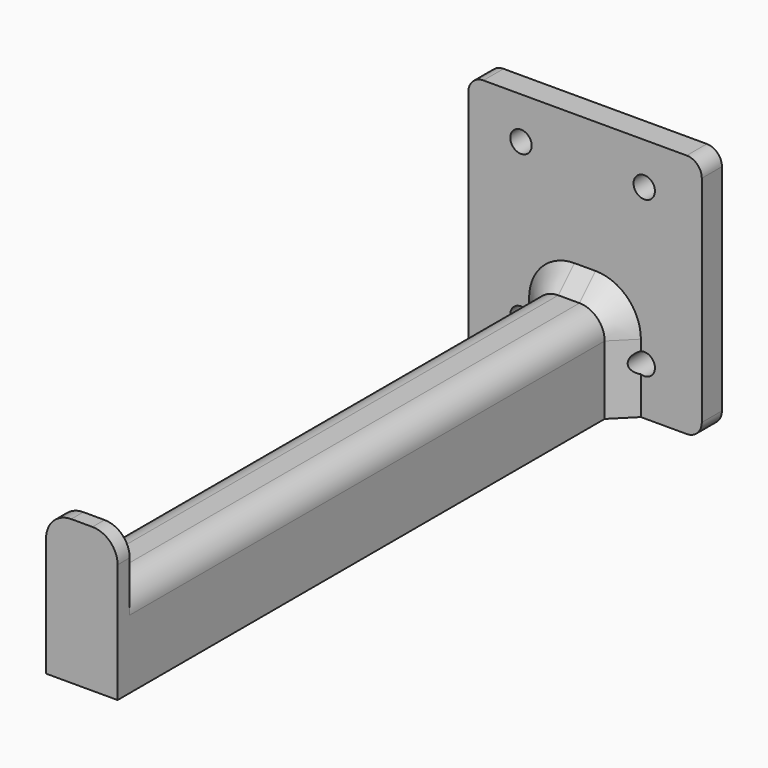
from build123d import *

# Parameters (mm, degrees)
F0_R         = 2.1251138046
F1_DEPTH     = 5
F0_W         = 14.2144468555
F0_H         = 18.6405025888
F2_DEPTH     = 130
F3_W         = 14.2144468555
F3_H         = 3
F4_DEPTH     = 10.03026
F5_R         = 5
F6_R         = 3
F7_T1_DEPTH  = 4.2144468555
F7_T6_DEPTH  = 13.6405025888
F7_S7_R      = 2.1251138046
F7_T8_DEPTH  = 9
F7_T10_ANGLE = 90
F7_T12_ANGLE = 90
F7_T16_DEPTH = 13.6405025888
F7_S17_R     = 2.1251138046
F7_T18_DEPTH = 9


# Not quite as in the source:
# - a fillet or chamfer that OpenCascade refuses, or shapes differently, is made with other operations: its cross-section is extruded or revolved along the edge and cut away or added


with BuildPart() as f1:
    # F0 (on Front) → F1 (new body)
    with BuildSketch(Plane.XZ):
        Polygon((16.5932904929, 31.273946166), (-29.8148933798, 31.273946166), (-29.8148933798, -17.4539741129), (-13.7278847396, -17.4539741129), (-13.7278847396, 1.186528476), (0.4865621158, 1.186528476), (0.4865621158, -17.4539741129), (16.5932904929, -17.4539741129), align=None)
        with Locations((-19.3455703557, -7.9430211366)):
            Circle(F0_R, mode=Mode.SUBTRACT)
        with Locations((5.1544296443, -7.9430211366)):
            Circle(F0_R, mode=Mode.SUBTRACT)
        with Locations((-19.3455703557, 22.9763388634)):
            Circle(F0_R, mode=Mode.SUBTRACT)
        with Locations((5.1544296443, 22.9763388634)):
            Circle(F0_R, mode=Mode.SUBTRACT)
    extrude(amount=F1_DEPTH)

    # F0 (on Front) → F2 (join)
    with BuildSketch(Plane.XZ):
        with Locations((-6.6206613119, -8.1337228185)):
            Rectangle(F0_W, F0_H)
    extrude(amount=F2_DEPTH)

    # F3 (on face) → F4 (join)
    with BuildSketch(Plane.XY.offset(1.186528476)):
        with Locations((-6.6206613119, -128.5)):
            Rectangle(F3_W, F3_H)
    extrude(amount=F4_DEPTH)

    # F5
    f5_edges = [f1.edges().sort_by_distance(p)[0] for p in [
        (0.486562, -66, 1.186528),
        (-13.727885, -66, 1.186528),
        (-13.727885, -128.5, 11.216788),
        (0.486562, -128.5, 11.216788),
    ]]
    fillet(f5_edges, radius=F5_R)

    # F6
    f6_edges = [f1.edges().sort_by_distance(p)[0] for p in [
        (-29.814893, -2.5, 31.273946),
        (16.59329, -2.5, 31.273946),
        (-29.814893, -2.5, -17.453974),
        (16.59329, -2.5, -17.453974),
    ]]
    fillet(f6_edges, radius=F6_R)

    # F7: chamfer of 4 on 2 edges, made by hand

    # F7_s2 → F7_t1 (join)
    with BuildSketch(Plane.YZ.offset(-8.7278847396)):
        Polygon((-5, 5.186528476), (-9, 1.186528476), (-5, 1.186528476), align=None)
    extrude(amount=F7_T1_DEPTH)


with BuildPart() as f7_tool4:
    # F7_s5 → F7_t6 (new body)
    with BuildSketch(Plane.XY.offset(-3.813471524)):
        Polygon((4.4865621158, -5), (0.4865621158, -9), (0.4865621158, -5), align=None)
    extrude(amount=-F7_T6_DEPTH)

    # F7_s7 → F7_t8 (cut, symmetric)
    with BuildSketch(Plane.XZ.offset(7)):
        with Locations((5.1544296443, -7.9430211366)):
            Circle(F7_S7_R)
    extrude(amount=F7_T8_DEPTH, both=True, mode=Mode.SUBTRACT)


with BuildPart() as f1_1:
    add(f1.part)

    # F7_t3: union F7_tool4
    add(f7_tool4.part)

    # F7_s9 → F7_t10 (revolve)
    with BuildSketch(Plane.XY.offset(-3.813471524)):
        Polygon((4.4865621158, -5), (0.4865621158, -9), (0.4865621158, -5), align=None)
    revolve(axis=Axis((-4.5134378842, -5, -3.813471524), (0, -1, 0)), revolution_arc=F7_T10_ANGLE)

    # F7_s11 → F7_t12 (revolve)
    with BuildSketch(Plane.YZ.offset(-8.7278847396)):
        Polygon((-5, 5.186528476), (-9, 1.186528476), (-5, 1.186528476), align=None)
    revolve(axis=Axis((-8.7278847396, -5, -3.813471524), (0, -1, 0)), revolution_arc=F7_T12_ANGLE)


with BuildPart() as f7_tool14:
    # F7_s15 → F7_t16 (new body)
    with BuildSketch(Plane.XY.offset(-17.4539741129)):
        Polygon((-17.7278847396, -5), (-13.7278847396, -9), (-13.7278847396, -5), align=None)
    extrude(amount=F7_T16_DEPTH)

    # F7_s17 → F7_t18 (cut, symmetric)
    with BuildSketch(Plane.XZ.offset(7)):
        with Locations((-19.3455703557, -7.9430211366)):
            Circle(F7_S17_R)
    extrude(amount=F7_T18_DEPTH, both=True, mode=Mode.SUBTRACT)


with BuildPart() as f1_2:
    add(f1_1.part)

    # F7_t13: union F7_tool14
    add(f7_tool14.part)


solid = f1_2.part
